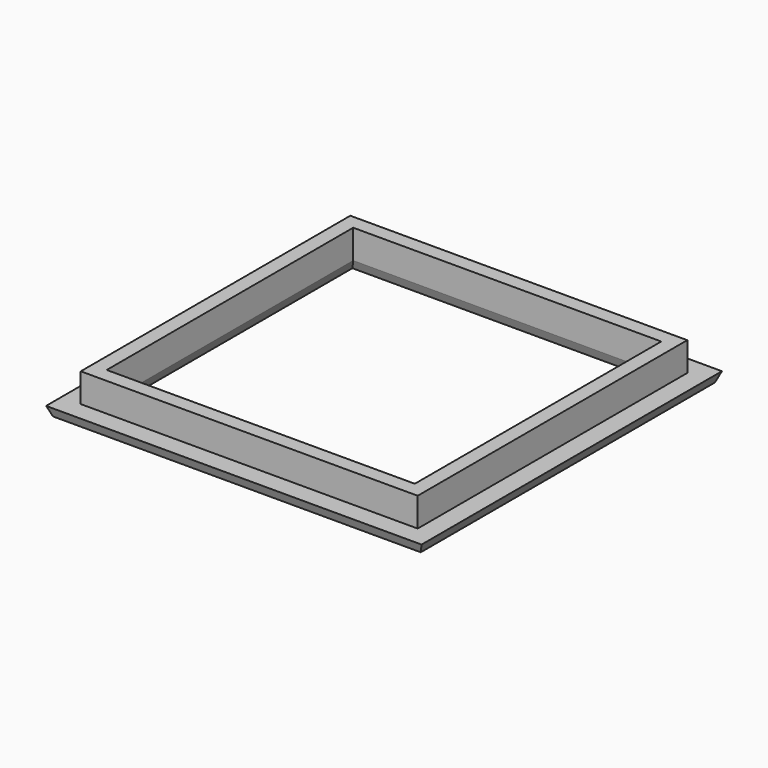
from build123d import *

# Parameters (mm, degrees)
F0_W     = 35
F0_H     = 35
F0_W_2   = 32
F0_H_2   = 32
F1_DEPTH = 4
F0_W_3   = 39
F0_H_3   = 39
F2_DEPTH = 1
F3_SIZE2 = 0.99999
F3_SIZE  = 0.39999


# Not quite as in the source:
# - a fillet or chamfer is up to 0.001 mm smaller than in the source, because OpenCascade refuses the exact size


with BuildPart() as f1:
    # F0 (on Top) → F1 (new body)
    with BuildSketch(Plane.XY):
        Rectangle(F0_W, F0_H)
        Rectangle(F0_W_2, F0_H_2, mode=Mode.SUBTRACT)
    extrude(amount=F1_DEPTH)

    # F0 (on Top) → F2 (join)
    with BuildSketch(Plane.XY):
        Rectangle(F0_W_3, F0_H_3)
        Rectangle(F0_W, F0_H, mode=Mode.SUBTRACT)
    extrude(amount=F2_DEPTH)

    # F3 (size 0.4 and 1 in the source; OpenCascade refuses exactly that, so slightly less here)
    f3_edges = [f1.edges().sort_by_distance(p)[0] for p in [
        (0, -19.5, 0),
        (19.5, 0, 0),
        (0, 19.5, 0),
        (-19.5, 0, 0),
        (-16, 0, 0),
        (0, 16, 0),
        (16, 0, 0),
        (0, -16, 0),
    ]]
    f3_side = f1.faces().sort_by_distance((0, -18.948457, 0))[0]
    chamfer(f3_edges, length=F3_SIZE, length2=F3_SIZE2, reference=f3_side)


solid = f1.part
